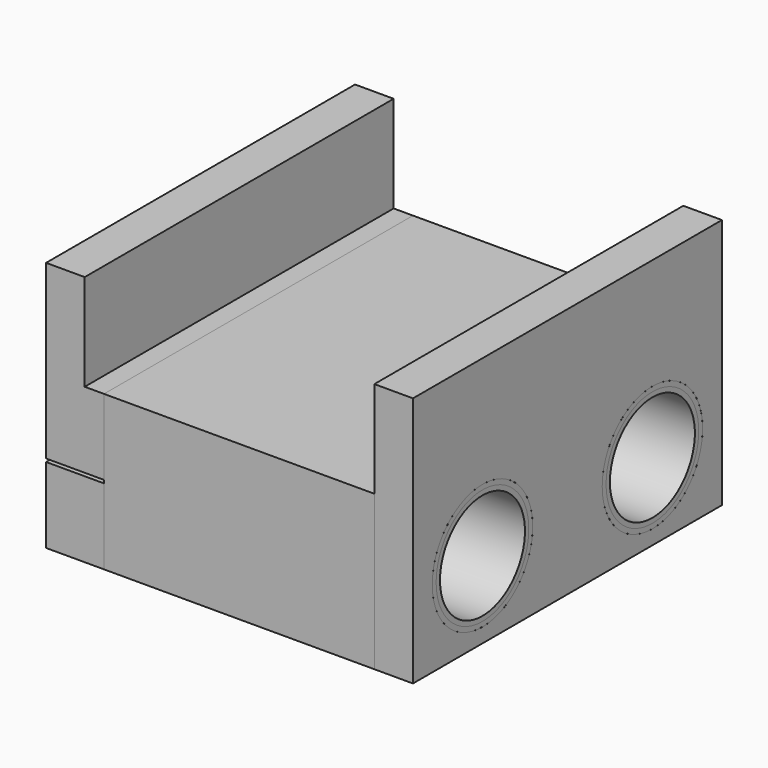
from build123d import *

# Parameters (mm, degrees)
F0_W          = 127
F0_H          = 50.8
F0_R          = 20.6375
F1_DEPTH      = 88.9
F2_R          = 20.6375
F2_R_2        = 19.05
F3_DEPTH      = 101.6
F4_DEPTH      = 12.7
F5_DEPTH      = 31.75
F6_R          = 19.05
F6_R_2        = 17.4625
F7_DEPTH      = 101.6
F7_DEPTH_BACK = 19.05
F9_DEPTH      = 19.05
F10_W         = 6.35
F10_H         = 127
F11_DEPTH     = 31.75
F12_R         = 17.4625
F13_DEPTH     = 76.2
F15_DEPTH     = 12.7
F16_R         = 3.175
F17_DEPTH     = 22.225
F18_R         = 14.2875
F19_DEPTH     = 44.45


with BuildPart() as f1:
    # F0 (on Right) → F1 (new body)
    with BuildSketch(Plane.YZ):
        with Locations((63.5, 25.4)):
            Rectangle(F0_W, F0_H)
        with Locations((28.575, 25.4)):
            Circle(F0_R, mode=Mode.SUBTRACT)
        with Locations((98.425, 25.4)):
            Circle(F0_R, mode=Mode.SUBTRACT)
    extrude(amount=F1_DEPTH)


with BuildPart() as f3:
    # F2 (on face) → F3 (new body)
    with BuildSketch(Plane(origin=(0, 0, 0), x_dir=(0, -1, 0), z_dir=(-1, 0, 0))):
        with Locations((-98.425, 25.4)):
            Circle(F2_R)
        with Locations((-98.425, 25.4)):
            Circle(F2_R_2, mode=Mode.SUBTRACT)
    extrude(amount=-F3_DEPTH)


with BuildPart() as f3b:
    # F2 (on face) → F3, piece 2 (new body)
    with BuildSketch(Plane(origin=(0, 0, 0), x_dir=(0, -1, 0), z_dir=(-1, 0, 0))):
        with Locations((-28.575, 25.4)):
            Circle(F2_R)
        with Locations((-28.575, 25.4)):
            Circle(F2_R_2, mode=Mode.SUBTRACT)
    extrude(amount=-F3_DEPTH)


with BuildPart() as f4:
    # F4 (new): a face of the model
    f4_faces = [f1.part.faces().sort_by_distance(p)[0] for p in [
        (88.9, 63.5, 25.4),
    ]]
    extrude(f4_faces, amount=F4_DEPTH)

    # F5 (add): a face of the model
    f5_faces = [f4.faces().sort_by_distance(p)[0] for p in [
        (95.25, 63.5, 50.8),
    ]]
    extrude(f5_faces, amount=F5_DEPTH)


with BuildPart() as f7:
    # F6 (on face) → F7 (new body, two sides)
    with BuildSketch(Plane(origin=(0, 0, 0), x_dir=(0, -1, 0), z_dir=(-1, 0, 0))) as f7_sk:
        with Locations((-98.425, 25.4)):
            Circle(F6_R)
        with Locations((-98.425, 25.4)):
            Circle(F6_R_2, mode=Mode.SUBTRACT)
    extrude(amount=-F7_DEPTH)
    extrude(f7_sk.sketch, amount=F7_DEPTH_BACK)


with BuildPart() as f7b:
    # F6 (on face) → F7, piece 2 (new body, two sides)
    with BuildSketch(Plane(origin=(0, 0, 0), x_dir=(0, -1, 0), z_dir=(-1, 0, 0))) as f7_2_sk:
        with Locations((-28.575, 25.4)):
            Circle(F6_R)
        with Locations((-28.575, 25.4)):
            Circle(F6_R_2, mode=Mode.SUBTRACT)
    extrude(amount=-F7_DEPTH)
    extrude(f7_2_sk.sketch, amount=F7_DEPTH_BACK)


with BuildPart() as f9:
    # F8 (on face) → F9 (new body)
    with BuildSketch(Plane(origin=(0, 0, 0), x_dir=(0, -1, 0), z_dir=(-1, 0, 0))):
        with BuildLine():
            Line((-127, 24.892), (-127, 0))
            Line((-127, 0), (0, 0))
            Line((0, 0), (0, 24.892))
            Line((0, 24.892), (-9.5317745379, 24.892))
            ThreePointArc((-9.5317745379, 24.892), (-47.625, 25.4), (-9.5317745379, 25.908))
            Line((-9.5317745379, 25.908), (0, 25.908))
            Line((0, 25.908), (0, 82.55))
            Line((0, 82.55), (-127, 82.55))
            Line((-127, 82.55), (-127, 25.908))
            Line((-127, 25.908), (-117.4682254621, 25.908))
            ThreePointArc((-117.4682254621, 25.908), (-79.375, 25.4), (-117.4682254621, 24.892))
            Line((-117.4682254621, 24.892), (-127, 24.892))
        make_face()
    extrude(amount=F9_DEPTH)

    # F10 (on face) → F11 (cut)
    with BuildSketch(Plane.XY.offset(82.55)):
        with Locations((-3.175, 63.5)):
            Rectangle(F10_W, F10_H)
    extrude(amount=-F11_DEPTH, mode=Mode.SUBTRACT)


with BuildPart() as f13:
    # F12 (on face) → F13 (new body)
    with BuildSketch(Plane(origin=(-19.05, 0, 0), x_dir=(0, -1, 0), z_dir=(-1, 0, 0))):
        with Locations((-98.425, 25.4)):
            Circle(F12_R)
    extrude(amount=-F13_DEPTH)


with BuildPart() as f13b:
    # F12 (on face) → F13, piece 2 (new body)
    with BuildSketch(Plane(origin=(-19.05, 0, 0), x_dir=(0, -1, 0), z_dir=(-1, 0, 0))):
        with Locations((-28.575, 25.4)):
            Circle(F12_R)
    extrude(amount=-F13_DEPTH)


with BuildPart() as f15_tool:
    # F14 (on face) → F15 (new body)
    with BuildSketch(Plane(origin=(0, 0, 0), x_dir=(1, 0, 0), z_dir=(0, 0, -1))):
        with BuildLine():
            Line((5.842, -31.877), (44.45, -31.877))
            ThreePointArc((44.45, -31.877), (47.752, -28.575), (44.45, -25.273))
            Line((44.45, -25.273), (5.842, -25.273))
            ThreePointArc((5.842, -25.273), (2.54, -28.575), (5.842, -31.877))
        make_face()
        with BuildLine():
            Line((5.842, -101.727), (44.45, -101.727))
            ThreePointArc((44.45, -101.727), (47.752, -98.425), (44.45, -95.123))
            Line((44.45, -95.123), (5.842, -95.123))
            ThreePointArc((5.842, -95.123), (2.54, -98.425), (5.842, -101.727))
        make_face()
    extrude(amount=-F15_DEPTH)


with BuildPart() as f7_1:
    add(f7.part)

    # F15: cut by f15_tool
    add(f15_tool.part, mode=Mode.SUBTRACT)


with BuildPart() as f7b_1:
    add(f7b.part)

    # F15: cut by f15_tool
    add(f15_tool.part, mode=Mode.SUBTRACT)


with BuildPart() as f17_tool:
    # F16 (on face) → F17 (new body)
    with BuildSketch(Plane(origin=(0, 0, 0), x_dir=(1, 0, 0), z_dir=(0, 0, -1))):
        with Locations((5.842, -98.425)):
            Circle(F16_R)
        with Locations((5.842, -28.575)):
            Circle(F16_R)
    extrude(amount=-F17_DEPTH)


with BuildPart() as f1_1:
    add(f1.part)

    # F17: cut by f17_tool
    add(f17_tool.part, mode=Mode.SUBTRACT)


with BuildPart() as f3_1:
    add(f3.part)

    # F17: cut by f17_tool
    add(f17_tool.part, mode=Mode.SUBTRACT)


with BuildPart() as f3b_1:
    add(f3b.part)

    # F17: cut by f17_tool
    add(f17_tool.part, mode=Mode.SUBTRACT)


with BuildPart() as f13_1:
    add(f13.part)

    # F17: cut by f17_tool
    add(f17_tool.part, mode=Mode.SUBTRACT)


with BuildPart() as f13b_1:
    add(f13b.part)

    # F17: cut by f17_tool
    add(f17_tool.part, mode=Mode.SUBTRACT)


with BuildPart() as f19_tool:
    # F18 (on face) → F19 (new body)
    with BuildSketch(Plane.YZ.offset(57.15)):
        with Locations((98.425, 25.4)):
            Circle(F18_R)
        with Locations((28.575, 25.4)):
            Circle(F18_R)
    extrude(amount=-F19_DEPTH)


with BuildPart() as f13_2:
    add(f13_1.part)

    # F19: cut by f19_tool
    add(f19_tool.part, mode=Mode.SUBTRACT)


with BuildPart() as f13b_2:
    add(f13b_1.part)

    # F19: cut by f19_tool
    add(f19_tool.part, mode=Mode.SUBTRACT)


solid = Compound([f4.part, f9.part, f7_1.part, f7b_1.part, f1_1.part, f3_1.part, f3b_1.part, f13_2.part, f13b_2.part])
